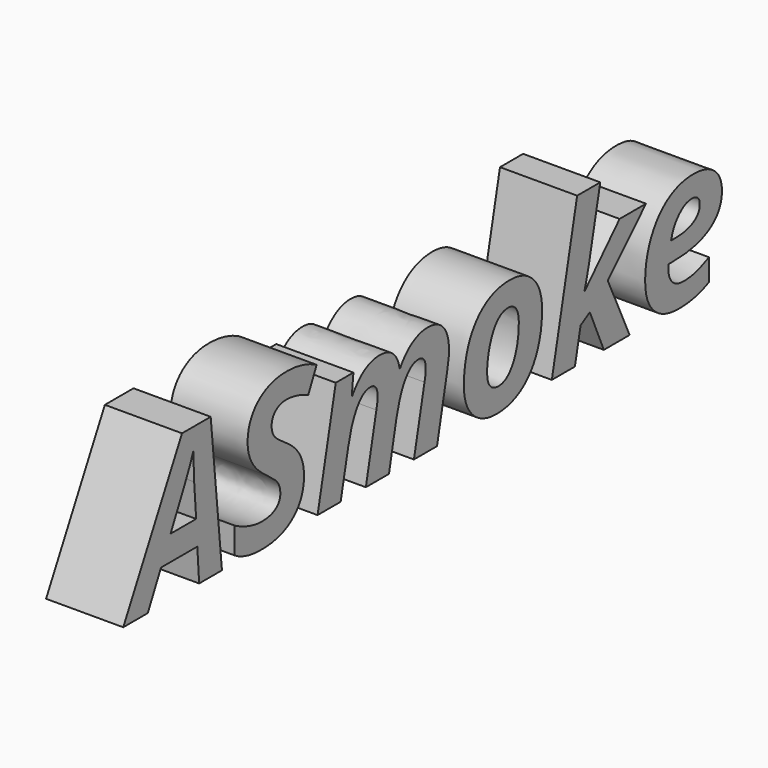
from build123d import *

# Parameters (mm, degrees)
F0_TEXT_SIZE = 63.677980668
F1_DEPTH     = 25


# Not quite as in the source:
# - Text() gives the source's letters only with a copy of the font that has no kerning and outlines rounded to 1/6400 em; it was checked with that copy


with BuildPart() as f1:
    # F0 (on Right) → F1 (new body)
    with BuildSketch(Plane.YZ):
        with Locations((-83.1935927272, -7.502399385)):
            Text('ASmoke', F0_TEXT_SIZE, font='Open Sans', font_style=FontStyle.BOLDITALIC, text_align=(TextAlign.LEFT, TextAlign.BOTTOM))
    extrude(amount=F1_DEPTH)


solid = f1.part
